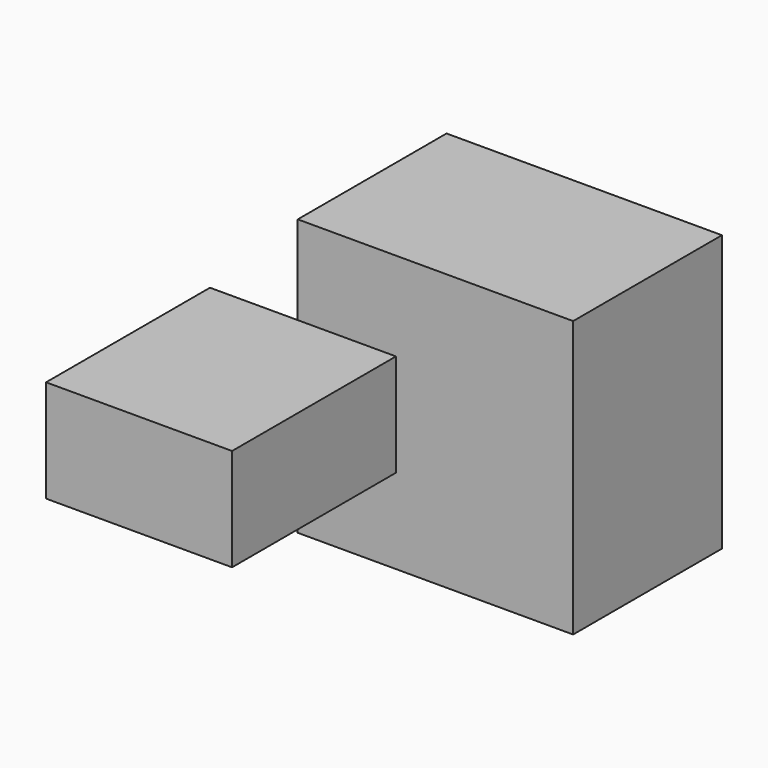
from build123d import *

# Parameters (mm, degrees)
F1_DEPTH = 25
F2_W     = 27.5361537933
F2_H     = 13.7671530247
F3_DEPTH = 25


# Not quite as in the source:
# - a feature names something its author has since deleted; it is built from what else it names


with BuildPart() as f1:
    # F0 (on Front) → F1 (new body)
    with BuildSketch(Plane.XZ):
        Polygon((37.0171777904, 0), (37.0171777904, 37.0931364596), (0, 37.0931364596), (0, 18.5465682298), (0, 0), align=None)
    extrude(amount=F1_DEPTH)


with BuildPart() as f3:
    # F2 (on Right) → F3 (new body)
    with BuildSketch(Plane.YZ):
        with Locations((-53.5176098347, 28.1172171235)):
            Rectangle(F2_W, F2_H)
    extrude(amount=F3_DEPTH)


solid = Compound([f1.part, f3.part])
